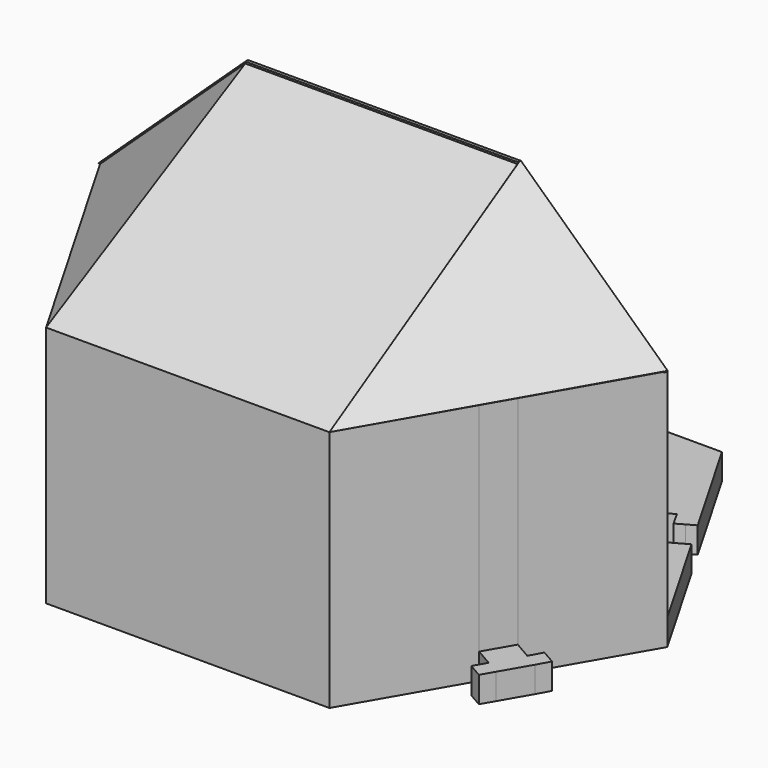
from build123d import *

# Parameters (mm, degrees)
F0_W      = 50
F0_H      = 12.5
F1_DEPTH  = 8
F2_DEPTH  = 75
F4_DEPTH  = 8
F7_DEPTH  = 3
F8_DEPTH  = 1
F11_DEPTH = 3
F14_DEPTH = 3
F15_DEPTH = 8
F16_DEPTH = 8
F17_DEPTH = 8
F18_DEPTH = 8


# Not quite as in the source:
# - a feature names something its author has since deleted; it is built from what else it names


with BuildPart() as f1:
    # F0 (on Top) → F1 (new body)
    with BuildSketch(Plane.XY):
        Polygon((-42.0179491924, 72.7772228311), (-60.5095952989, 40.7487522591), (-57.9695070384, 39.3207329262), (-55.5194165334, 43.6791064608), (-50.2642610162, 40.7248836223), (-52.7144317239, 36.366367418), (-57.615009792, 27.6494680496), (-60.0654171506, 23.2910848888), (-65.3204122546, 26.2455930623), (-62.870004896, 30.6039762231), (-65.5097997054, 32.0881441788), (-84.0358983849, 0), (-42.0179491924, -72.7772228311), (42.0179491924, -72.7772228311), (84.0358983849, 0), (65.5097997054, 32.0881441788), (62.870004896, 30.6039762231), (65.3204122546, 26.2455930623), (60.0654171506, 23.2910848888), (57.615009792, 27.6494680496), (55.164720758, 32.0079177338), (52.7144317239, 36.366367418), (50.2642610162, 40.7248836223), (55.5194165334, 43.6791064608), (57.9695070384, 39.3207329262), (60.5095952989, 40.7487522591), (42.0179491924, 72.7772228311), align=None)
        with Locations((0, 54.5829171234)):
            Rectangle(F0_W, F0_H, mode=Mode.SUBTRACT)
    extrude(amount=F1_DEPTH)

    # F0 (on Top) → F2 (join)
    with BuildSketch(Plane.XY):
        Polygon((68.1424599038, -33.5282429562), (87.5, 0), (84.0358983849, 0), (42.0179491924, -72.7772228311), (-42.0179491924, -72.7772228311), (-84.0358983849, 0), (-87.5, 0), (-43.75, -75.7772228311), (43.75, -75.7772228311), (63.1424599038, -42.188496994), align=None)
    extrude(amount=F2_DEPTH)

    # F0 (on Top) → F4 (join)
    with BuildSketch(Plane.XY):
        Polygon((43.75, 75.7772228311), (-43.75, 75.7772228311), (-63.1248363216, 42.2190219338), (-60.5095952989, 40.7487522591), (-42.0179491924, 72.7772228311), (42.0179491924, 72.7772228311), (60.5095952989, 40.7487522591), (63.1248363216, 42.2190219338), align=None)
    extrude(amount=F4_DEPTH)

    # F6 (on face) → F7 (join)
    with BuildSketch(Plane(origin=(0, -50.1312366318, 89.3836679776), x_dir=(1, 0, 0), z_dir=(0, 0.4891706574, -0.872188092))):
        Polygon((43.75, 29.4041920927), (0, 29.4041920927), (-43.75, 29.4041920927), (-42.01795, -57.4775522498), (42.01795, -57.4775522498), align=None)
    extrude(amount=F7_DEPTH)

    # F3 (on Front) → F8 (join)
    with BuildSketch(Plane.XZ):
        Polygon((-42.01795, 114.5), (0, 114.5), (42.01795, 114.5), (84.0359, 75), (87.5, 75), (42.01795, 117.5), (0, 117.5), (-42.01795, 117.5), (-87.5, 75), (-84.0359, 75), align=None)
    extrude(amount=F8_DEPTH)

    # F10 (on face) → F11 (join)
    with BuildSketch(Plane(origin=(-67.6846727043, -39.0777640058, 72.4338274863), x_dir=(0.7723629594, -0.3015876344, 0.5590173143), z_dir=(-0.6351814378, -0.3667221741, 0.6797495039))):
        Polygon((33.2314262259, 55.789645187), (-25.6554603702, 35.6104118215), (30.9888924807, -31.0804218073), align=None)
    extrude(amount=-F11_DEPTH)

    # F13 (on face) → F14 (join)
    with BuildSketch(Plane(origin=(67.6756688636, -39.5950852503, 72.4241918832), x_dir=(0.7733047167, 0.3041472681, -0.556322078), z_dir=(-0.6340345536, 0.3709553614, -0.6785221475))):
        Polygon((-30.939509805, 30.5117392321), (-32.8751652468, -56.3649154418), (25.9400068576, -35.9776056011), align=None)
    extrude(amount=F14_DEPTH)

    # F0 (on Top) → F15 (join)
    with BuildSketch(Plane.XY):
        with Locations((0, 54.5829171234)):
            Rectangle(F0_W, F0_H)
    extrude(amount=F15_DEPTH)

    # F0 (on Top) → F16 (join)
    with BuildSketch(Plane.XY):
        Polygon((75.7376143812, -32.7192219692), (73.5984199476, -36.6782429562), (77.9285469666, -39.1782429562), (80.1153549422, -35.2453215385), align=None)
        Polygon((73.5984199476, -36.6782429562), (68.1424599038, -33.5282429562), (63.1424599038, -42.188496994), (68.5982950526, -45.3387133087), (72.9283229484, -47.838884987), (77.9285469666, -39.1782429562), align=None)
        Polygon((72.9283229484, -47.838884987), (68.5982950526, -45.3387133087), (66.3481405421, -49.235738415), (70.6781684379, -51.7359100933), align=None)
    extrude(amount=F16_DEPTH)

    # F0 (on Top) → F17 (join)
    with BuildSketch(Plane.XY):
        Polygon((-65.5097997054, 32.0881441788), (-68.125, 33.5584843966), (-87.5, 0), (-84.0358983849, 0), align=None)
    extrude(amount=F17_DEPTH)

    # F0 (on Top) → F18 (join)
    with BuildSketch(Plane.XY):
        Polygon((87.5, 0), (68.125, 33.5584843966), (65.5097997054, 32.0881441788), (84.0358983849, 0), align=None)
    extrude(amount=F18_DEPTH)


solid = f1.part
